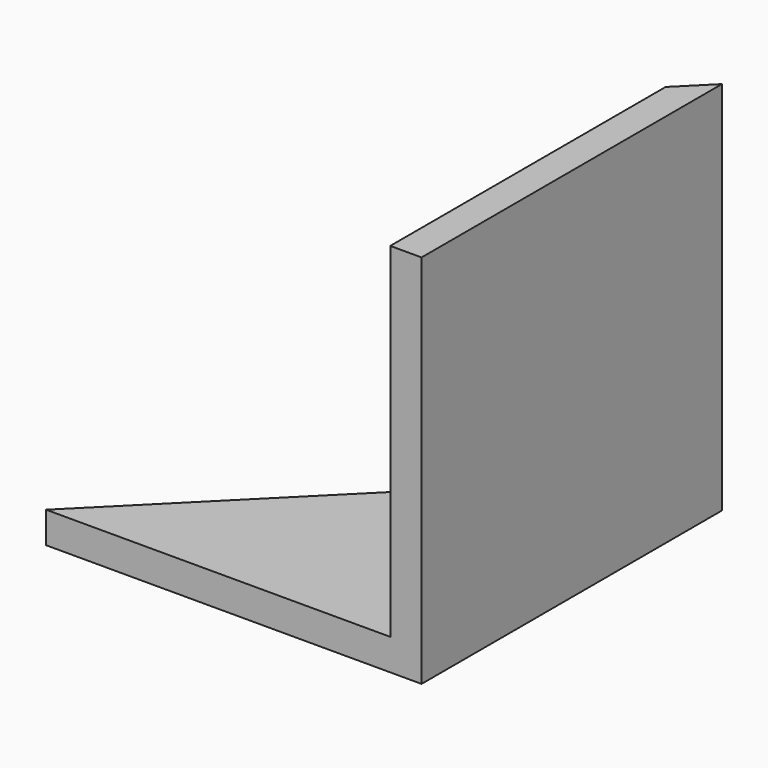
from build123d import *

# Parameters (mm, degrees)
F1_DEPTH = 76.2
F3_DEPTH = 38.101


# Not quite as in the source:
# - a feature names something its author has since deleted; it is built from what else it names


with BuildPart() as f1:
    # F0 (on Front) → F1 (new body)
    with BuildSketch(Plane.XZ):
        Polygon((0, 3.175), (0, 0), (38.1, 0), (38.1, 38.1), (34.925, 38.1), (34.925, 3.175), align=None)
    extrude(amount=F1_DEPTH)

    # F2 (on face) → F3 (cut, through all)
    with BuildSketch(Plane.XY.offset(38.1)):
        Polygon((34.925, -41.275), (34.925, 0), (0, 0), (0, -76.2), align=None)
        Polygon((38.1, 0), (34.925, 0), (34.925, -41.275), (38.1, -38.1), align=None)
    extrude(amount=-F3_DEPTH, mode=Mode.SUBTRACT)


solid = f1.part
